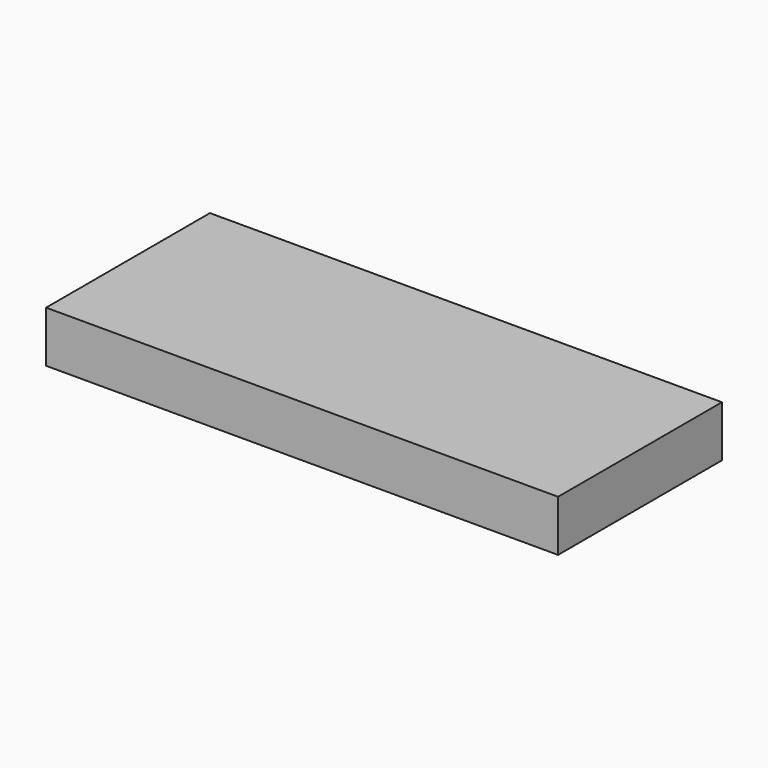
from build123d import *

# Parameters (mm, degrees)
F1_DEPTH = 2.5


# Not quite as in the source:
# - a feature names something its author has since deleted; it is built from what else it names


with BuildPart() as f1:
    # F0 (on Top) → F1 (new body, symmetric)
    with BuildSketch(Plane.XY):
        Polygon((-50, 0), (0, 0), (0, 20), (-50, 20), (-50, 10), align=None)
    extrude(amount=F1_DEPTH, both=True)


solid = f1.part
